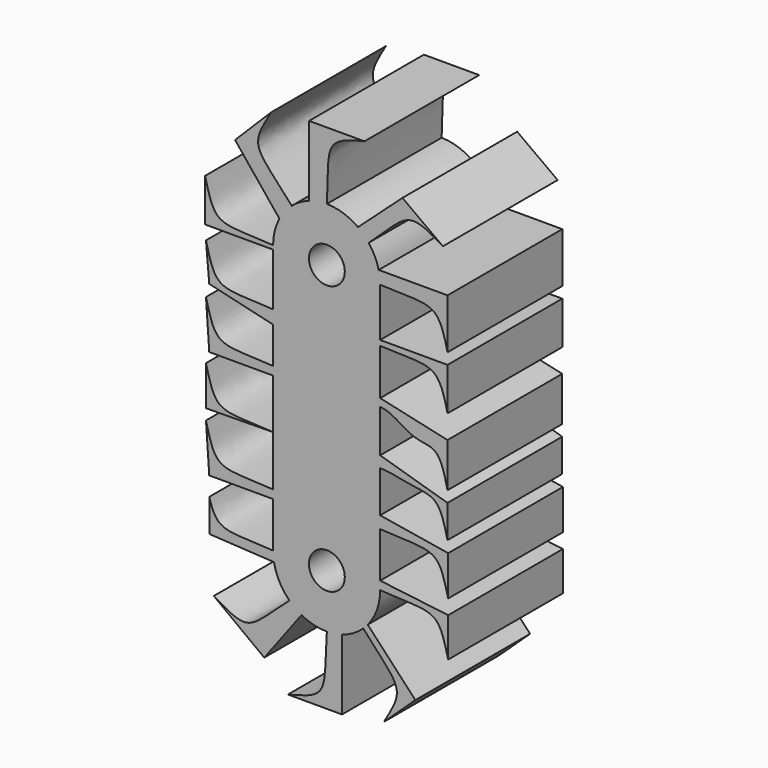
from build123d import *

# Parameters (mm, degrees)
F0_R     = 6.35
F1_DEPTH = 50.8


# Not quite as in the source:
# - ends of sketch curves that miss each other by under 0.0002 mm in the source are joined


with BuildPart() as f1:
    # F0 (on Front) → F1 (new body)
    with BuildSketch(Plane.XZ):
        with BuildLine():
            ThreePointArc((0, 66.6748002519), (-0.0436185803, 66.6749500629), (-0.0872373893, 66.675))
            Line((-0.0872373893, 66.675), (0.0872373893, 66.675))
            add(Edge.make_bspline(
                [(0.0872373857, 66.675), (0.2430286091, 70.7234059267), (0.2508794322, 78.1359164956), (1.3441036555, 87.6367445855), (9.1396162432, 89.5194059267), (13.3915788725, 90.5324317255)],
                knots=[0, 0, 0, 0, 0.3552568963, 0.6495702629, 1, 1, 1, 1], degree=3))
            Line((13.3915788725, 90.5324317255), (-6.2023079954, 90.5324317255))
            Line((-6.2023079954, 90.5324317255), (-6.2023079954, 65.6067718497))
            ThreePointArc((-6.2023079954, 65.6067718497), (-3.1455649251, 66.398691411), (0, 66.6748002519))
        make_face()
        with BuildLine():
            Line((0.0872373893, 66.675), (-0.0872373893, 66.675))
            ThreePointArc((-0.0872373893, 66.675), (-0.0436185803, 66.6749500629), (0, 66.6748002519))
            ThreePointArc((0, 66.6748002519), (0.0436185803, 66.6749500629), (0.0872373893, 66.675))
        make_face()
        with BuildLine():
            ThreePointArc((11.1189951284, 63.0302865199), (5.8462468924, 65.7273828343), (0, 66.6748002519))
            ThreePointArc((0, 66.6748002519), (-3.1455649251, 66.398691411), (-6.2023079954, 65.6067718497))
            ThreePointArc((-6.2023079954, 65.6067718497), (-9.4495187485, 64.1159909456), (-12.3612291686, 62.0450617321))
            ThreePointArc((-12.3612291686, 62.0450617321), (-14.7898940453, 59.5234646185), (-16.7160906478, 56.600002333))
            ThreePointArc((-16.7160906478, 56.600002333), (-18.3925610283, 52.2509648125), (-18.9627626107, 47.625))
            Line((-18.9627626107, 47.625), (-18.9627626107, 46.238899231))
            Line((-18.9627626107, 46.238899231), (-18.9627626107, 27.6209915512))
            Line((-18.9627626107, 27.6209915512), (-18.9627626107, 22.8571407497))
            Line((-18.9627626107, 22.8571407497), (-18.9627626107, 9.9559536659))
            Line((-18.9627626107, 9.9559536659), (-18.9627626107, 6.9569204934))
            Line((-18.9627626107, 6.9569204934), (-18.9627626107, -10.6532565794))
            add(Edge.make_bspline(
                [(-18.6444241287, -10.6651281533), (-18.7506005412, -10.661180346), (-18.8567145999, -10.657223662), (-18.9627626107, -10.6532565794)],
                knots=[0, 0, 0, 0, 0.0091079643, 0.0091079643, 0.0091079643, 0.0091079643], degree=3))
            Line((-18.6444241287, -10.6651281533), (-18.9627626107, -10.6689278948))
            Line((-18.9627626107, -10.6689278948), (-18.9627626107, -28.536211024))
            Line((-18.9627626107, -28.536211024), (-18.9627626107, -31.5352441965))
            Line((-18.9627626107, -31.5352441965), (-18.9627626107, -47.6131283575))
            Line((-18.9627626107, -47.6131283575), (-18.9627626107, -47.625))
            ThreePointArc((-18.9627626107, -47.625), (-18.883010592, -49.366318905), (-18.6444222927, -51.0930578942))
            ThreePointArc((-18.6444222927, -51.0930578942), (-16.706364569, -56.6181881592), (-13.1818276234, -61.2937385552))
            ThreePointArc((-13.1818276234, -61.2937385552), (-11.1490506185, -63.0083784263), (-8.8973030522, -64.4232300572))
            ThreePointArc((-8.8973030522, -64.4232300572), (-4.5862709651, -66.0928320239), (0, -66.6748002519))
            ThreePointArc((0, -66.6748002519), (0.0402063893, -66.6745736982), (0.0804122108, -66.6742622852))
            ThreePointArc((0.0804122108, -66.6742622852), (2.7974683178, -66.4553205757), (5.4554608651, -65.8508332062))
            ThreePointArc((5.4554608651, -65.8508332062), (9.4693916223, -64.1044824535), (12.9787289686, -61.4880091659))
            ThreePointArc((12.9787289686, -61.4880091659), (13.7941569026, -60.6714321756), (14.5586451488, -59.8069795058))
            ThreePointArc((14.5586451488, -59.8069795058), (17.8279316352, -54.1018216607), (18.9627626107, -47.625))
            Line((18.9627626107, -47.625), (18.9627626107, -44.6413718164))
            Line((18.9627626107, -44.6413718164), (18.9627626107, -28.575))
            Line((18.9627626107, -28.575), (18.9627626107, -24.2739211984))
            Line((18.9627626107, -24.2739211984), (18.9627626107, -9.525))
            Line((18.9627626107, -9.525), (18.9627626107, -5.5678933859))
            Line((18.9627626107, -5.5678933859), (18.9627626107, 9.525))
            Line((18.9627626107, 9.525), (18.9627626107, 12.2702307999))
            Line((18.9627626107, 12.2702307999), (18.9627626107, 28.575))
            Line((18.9627626107, 28.575), (18.9627626107, 30.3942766041))
            Line((18.9627626107, 30.3942766041), (18.9627626107, 47.625))
            ThreePointArc((18.9627626107, 47.625), (18.830991044, 49.8617684162), (18.4374993091, 52.0675927401))
            ThreePointArc((18.4374993091, 52.0675927401), (17.0655606958, 55.9125821474), (14.9058863631, 59.376967501))
            ThreePointArc((14.9058863631, 59.376967501), (13.1391851128, 61.33500539), (11.1189951284, 63.0302865199))
        make_face()
        with Locations((0.0872373893, -47.625)):
            Circle(F0_R, mode=Mode.SUBTRACT)
        with Locations((0.0872373893, 47.625)):
            Circle(F0_R, mode=Mode.SUBTRACT)
        with BuildLine():
            Line((26.852209121, 77.2689878941), (11.1189951284, 63.0302865199))
            ThreePointArc((11.1189951284, 63.0302865199), (13.1391851128, 61.33500539), (14.9058863631, 59.376967501))
            add(Edge.make_bspline(
                [(14.9058863631, 59.376967501), (17.8787026773, 62.1294617543), (23.1256905365, 67.365346873), (30.6168167674, 73.3104205806), (37.460319182, 69.129403368), (41.1832282024, 66.8391291713)],
                knots=[0, 0, 0, 0, 0.3552568963, 0.6495702629, 1, 1, 1, 1], degree=3))
            Line((41.1832282024, 66.8391291713), (26.852209121, 77.2689878941))
        make_face()
        with BuildLine():
            ThreePointArc((-16.7160906478, 56.600002333), (-14.7898940453, 59.5234646185), (-12.3612291686, 62.0450617321))
            add(Edge.make_bspline(
                [(-12.3612291686, 62.0450617321), (-15.1748332393, 65.0759741908), (-20.1862585725, 70.5200649728), (-26.3903403692, 78.1445018545), (-21.8820939834, 84.9502715651), (-19.6493531041, 88.8288373426)],
                knots=[0, 0, 0, 0, 0.354508674, 0.649032011, 1, 1, 1, 1], degree=3))
            Line((-19.6493531041, 88.8288373426), (-32.4367880821, 76.0538205504))
            Line((-32.4367880821, 76.0538205504), (-16.7160906478, 56.600002333))
        make_face()
        with BuildLine():
            Line((42.8201943362, 52.0675927401), (18.4374993091, 52.0675927401))
            ThreePointArc((18.4374993091, 52.0675927401), (18.830991044, 49.8617684162), (18.9627626107, 47.625))
            add(Edge.make_bspline(
                [(18.9627626107, 47.625), (23.0111685374, 47.4692087767), (30.4236791063, 47.4613579536), (39.9245071963, 46.3681337303), (41.8071685374, 38.5726211425), (42.8201943362, 34.3206585132)],
                knots=[0, 0, 0, 0, 0.3552568963, 0.6495702629, 1, 1, 1, 1], degree=3))
            Line((42.8201943362, 34.3206585132), (42.8201943362, 52.0675927401))
        make_face()
        with BuildLine():
            Line((-18.9627626107, 46.238899231), (-18.9627626107, 47.625))
            add(Edge.make_bspline(
                [(-18.9627626107, 47.625), (-23.0954598814, 47.7786602348), (-30.4886262273, 48.0846009077), (-40.2668655585, 49.0889436199), (-41.8914598814, 57.0891611241), (-43.0552338276, 61.4105075031)],
                knots=[0, 0, 0, 0, 0.354508674, 0.649032011, 1, 1, 1, 1], degree=3))
            Line((-43.0552338276, 61.4105075031), (-43.0552338276, 46.238899231))
            Line((-43.0552338276, 46.238899231), (-18.9627626107, 46.238899231))
        make_face()
        with BuildLine():
            Line((42.8201943411, 30.3942766041), (18.9627626107, 30.3942766041))
            Line((18.9627626107, 30.3942766041), (18.9627626107, 28.575))
            add(Edge.make_bspline(
                [(18.9627626107, 28.575), (23.0111685371, 28.4192087694), (30.4236791135, 28.4113579415), (39.9245072271, 27.3181337496), (41.8071685371, 19.5226211283), (42.8201943411, 15.2706584996)],
                knots=[0, 0, 0, 0, 0.3552568963, 0.6495702629, 1, 1, 1, 1], degree=3))
            Line((42.8201943411, 15.2706584996), (42.8201943411, 30.3942766041))
        make_face()
        with BuildLine():
            Line((-18.9627626107, 22.8571407497), (-18.9627626107, 27.6209915512))
            add(Edge.make_bspline(
                [(-18.9627626107, 27.6209915512), (-22.9844140999, 27.7714349554), (-30.2593476001, 28.0778684026), (-39.9485270765, 29.0730635972), (-41.5731213994, 37.0732811015), (-42.7368953456, 41.3946274804)],
                knots=[0.0091079643, 0.0091079643, 0.0091079643, 0.0091079643, 0.354508674, 0.649032011, 1, 1, 1, 1], degree=3))
            Line((-42.7368953456, 41.3946274804), (-41.5731213994, 28.2001979076))
            Line((-41.5731213994, 28.2001979076), (-18.9627626107, 22.8571407497))
        make_face()
        with BuildLine():
            Line((42.8098751268, 6.9569204934), (18.9627626107, 12.2702307999))
            Line((18.9627626107, 12.2702307999), (18.9627626107, 9.525))
            add(Edge.make_bspline(
                [(18.9627626107, 9.525), (23.1314562939, 9.364778535), (30.0786708201, 2.6539069602), (39.9702454496, 3.9214789741), (41.8090278021, -4.5252336061), (42.8098751268, -8.7066759335)],
                knots=[0, 0, 0, 0, 0.3658024663, 0.6552973413, 1, 1, 1, 1], degree=3))
            Line((42.8098751268, -8.7066759335), (42.8098751268, 6.9569204934))
        make_face()
        with BuildLine():
            Line((-18.9627626107, 6.9569204934), (-18.9627626107, 9.9559536659))
            add(Edge.make_bspline(
                [(-18.9627626107, 9.9559536659), (-22.9844140999, 10.10639707), (-30.2593476001, 10.4128305173), (-39.9485270765, 11.4080257119), (-41.5731213994, 19.4082432162), (-42.7368953456, 23.7295895951)],
                knots=[0.0091079643, 0.0091079643, 0.0091079643, 0.0091079643, 0.354508674, 0.649032011, 1, 1, 1, 1], degree=3))
            Line((-42.7368953456, 23.7295895951), (-41.5731213994, 6.9569204934))
            Line((-41.5731213994, 6.9569204934), (-18.9627626107, 6.9569204934))
        make_face()
        with BuildLine():
            Line((42.8098751268, -12.6443654299), (18.9627626107, -5.5678933859))
            Line((18.9627626107, -5.5678933859), (18.9627626107, -9.525))
            add(Edge.make_bspline(
                [(18.9627626107, -9.525), (23.0256837277, -9.6811561541), (30.3753295074, -11.6802210009), (39.9266576959, -12.0508755513), (41.7943803202, -20.0312831228), (42.8098751268, -24.2739211984)],
                knots=[0, 0, 0, 0, 0.3565209338, 0.6502525899, 1, 1, 1, 1], degree=3))
            Line((42.8098751268, -24.2739211984), (42.8098751268, -12.6443654299))
        make_face()
        with BuildLine():
            add(Edge.make_bspline(
                [(-18.6444241287, -10.6651281533), (-18.7506005412, -10.661180346), (-18.8567145999, -10.657223662), (-18.9627626107, -10.6532565794)],
                knots=[0, 0, 0, 0, 0.0091079643, 0.0091079643, 0.0091079643, 0.0091079643], degree=3))
            Line((-18.9627626107, -10.6532565794), (-18.9627626107, -10.6689278948))
            Line((-18.9627626107, -10.6689278948), (-18.6444241287, -10.6651281533))
        make_face()
        with BuildLine():
            Line((-18.9627626107, -10.6689278948), (-18.9627626107, -10.6532565794))
            add(Edge.make_bspline(
                [(-18.9627626107, -10.6532565794), (-22.9844140999, -10.5028131753), (-30.2593476001, -10.1963797281), (-39.9485270765, -9.2011845334), (-41.5731213994, -1.2009670292), (-42.7368953456, 3.1203793498)],
                knots=[0.0091079643, 0.0091079643, 0.0091079643, 0.0091079643, 0.354508674, 0.649032011, 1, 1, 1, 1], degree=3))
            Line((-42.7368953456, 3.1203793498), (-42.7368953456, -10.9526999295))
            Line((-42.7368953456, -10.9526999295), (-18.9627626107, -10.6689278948))
        make_face()
        with BuildLine():
            Line((43.0552338738, -28.2348524779), (18.9627626107, -24.2739211984))
            Line((18.9627626107, -24.2739211984), (18.9627626107, -28.575))
            add(Edge.make_bspline(
                [(18.9627626107, -28.575), (23.0954598996, -28.7286602208), (30.4886262184, -29.0346008867), (40.2668655483, -30.0389436981), (41.8914598996, -38.0391608321), (43.0552338738, -42.3605071535)],
                knots=[0, 0, 0, 0, 0.3545086755, 0.6490320146, 1, 1, 1, 1], degree=3))
            Line((43.0552338738, -42.3605071535), (43.0552338738, -28.2348524779))
        make_face()
        with BuildLine():
            Line((-18.9627626107, -31.5352441965), (-18.9627626107, -28.536211024))
            add(Edge.make_bspline(
                [(-18.9627626107, -28.536211024), (-22.9844140999, -28.3857676199), (-30.2593476001, -28.0793341726), (-39.9485270765, -27.084138978), (-41.5731213994, -19.0839214737), (-42.7368953456, -14.7625750948)],
                knots=[0.0091079643, 0.0091079643, 0.0091079643, 0.0091079643, 0.354508674, 0.649032011, 1, 1, 1, 1], degree=3))
            Line((-42.7368953456, -14.7625750948), (-41.5731213994, -31.5352441965))
            Line((-41.5731213994, -31.5352441965), (-18.9627626107, -31.5352441965))
        make_face()
        with BuildLine():
            Line((43.0552338276, -47.5783012807), (18.9627626107, -44.6413718164))
            Line((18.9627626107, -44.6413718164), (18.9627626107, -47.625))
            add(Edge.make_bspline(
                [(18.9627626107, -47.625), (23.0954598814, -47.7786602348), (30.4886262273, -48.0846009077), (40.2668655585, -49.0889436199), (41.8914598814, -57.0891611241), (43.0552338276, -61.4105075031)],
                knots=[0, 0, 0, 0, 0.354508674, 0.649032011, 1, 1, 1, 1], degree=3))
            Line((43.0552338276, -61.4105075031), (43.0552338276, -47.5783012807))
        make_face()
        with BuildLine():
            Line((-18.9627626107, -47.625), (-18.9627626107, -47.6131283575))
            add(Edge.make_bspline(
                [(-18.9627626107, -47.6131283575), (-22.984413459, -47.4626849717), (-30.259346278, -47.156251522), (-38.7733625028, -46.2817597185), (-40.8056843428, -40.8850393206), (-41.5731195634, -38.2003750823)],
                knots=[0.0091080169, 0.0091080169, 0.0091080169, 0.0091080169, 0.354508674, 0.649032011, 0.8798185749, 0.8798185749, 0.8798185749, 0.8798185749], degree=3))
            Line((-41.5731195634, -38.2003750823), (-41.5731195634, -49.7814901173))
            Line((-41.5731195634, -49.7814901173), (-18.6444222927, -51.0930578942))
            ThreePointArc((-18.6444222927, -51.0930578942), (-18.883010592, -49.366318905), (-18.9627626107, -47.625))
        make_face()
        with BuildLine():
            Line((31.425178051, -77.8287127614), (14.5586451488, -59.8069795058))
            ThreePointArc((14.5586451488, -59.8069795058), (13.7941569026, -60.6714321756), (12.9787289686, -61.4880091659))
            add(Edge.make_bspline(
                [(12.9787289686, -61.4880091659), (15.7923330393, -64.5189216247), (20.8037583725, -69.9630124067), (27.0078401692, -77.5874492883), (22.4995937834, -84.3932189989), (20.2668529041, -88.2717847765)],
                knots=[0, 0, 0, 0, 0.354508674, 0.649032011, 1, 1, 1, 1], degree=3))
            Line((20.2668529041, -88.2717847765), (31.425178051, -77.8287127614))
        make_face()
        with BuildLine():
            ThreePointArc((-8.8973030522, -64.4232300572), (-11.1490506185, -63.0083784263), (-13.1818276234, -61.2937385552))
            add(Edge.make_bspline(
                [(-13.1818276234, -61.2937385552), (-16.2127400821, -64.1073426259), (-21.6568308642, -69.118767959), (-29.2812677458, -75.3228497557), (-36.0870374564, -70.81460337), (-39.9656032339, -68.5818624906)],
                knots=[0, 0, 0, 0, 0.354508674, 0.649032011, 1, 1, 1, 1], degree=3))
            Line((-39.9656032339, -68.5818624906), (-22.0917928964, -81.9996222854))
            Line((-22.0917928964, -81.9996222854), (-8.8973030522, -64.4232300572))
        make_face()
        with BuildLine():
            Line((5.4554608651, -90.7667335021), (5.4554608651, -65.8508332062))
            ThreePointArc((5.4554608651, -65.8508332062), (2.7974683178, -66.4553205757), (0.0804122108, -66.6742622852))
            add(Edge.make_bspline(
                [(0.0804122108, -66.6742622852), (0.0804030753, -66.6745079851), (0.0803939398, -66.6747536846), (0.0803848041, -66.6749993838)],
                knots=[0, 0, 0, 0, 2.10765e-05, 2.10765e-05, 2.10765e-05, 2.10765e-05], degree=3))
            add(Edge.make_bspline(
                [(0.0803848041, -66.6749993838), (-0.0732678944, -70.8074397221), (-0.3792098648, -78.2003319927), (-1.3835314091, -87.978365233), (-9.3837489133, -89.602959556), (-13.7050952923, -90.7667335021)],
                knots=[2.10765e-05, 2.10765e-05, 2.10765e-05, 2.10765e-05, 0.354508674, 0.649032011, 1, 1, 1, 1], degree=3))
            Line((-13.7050952923, -90.7667335021), (5.4554608651, -90.7667335021))
        make_face()
        with BuildLine():
            add(Edge.make_bspline(
                [(0.0804122108, -66.6742622852), (0.0804030753, -66.6745079851), (0.0803939398, -66.6747536846), (0.0803848041, -66.6749993838)],
                knots=[0, 0, 0, 0, 2.10765e-05, 2.10765e-05, 2.10765e-05, 2.10765e-05], degree=3))
            ThreePointArc((0.0804122108, -66.6742622852), (0.0402063893, -66.6745736982), (0, -66.6748002519))
            ThreePointArc((0, -66.6748002519), (0.0401922975, -66.6749419096), (0.0803848041, -66.6749993838))
        make_face()
        with BuildLine():
            ThreePointArc((0.0803848044, -66.6749987675), (0.0401922975, -66.6749419096), (0, -66.6748002519))
            ThreePointArc((0, -66.6748002519), (-0.0436185803, -66.6749500629), (-0.0872373893, -66.675))
            Line((-0.0872373893, -66.675), (0.0803848044, -66.6749987675))
        make_face()
    extrude(amount=F1_DEPTH)


solid = f1.part
